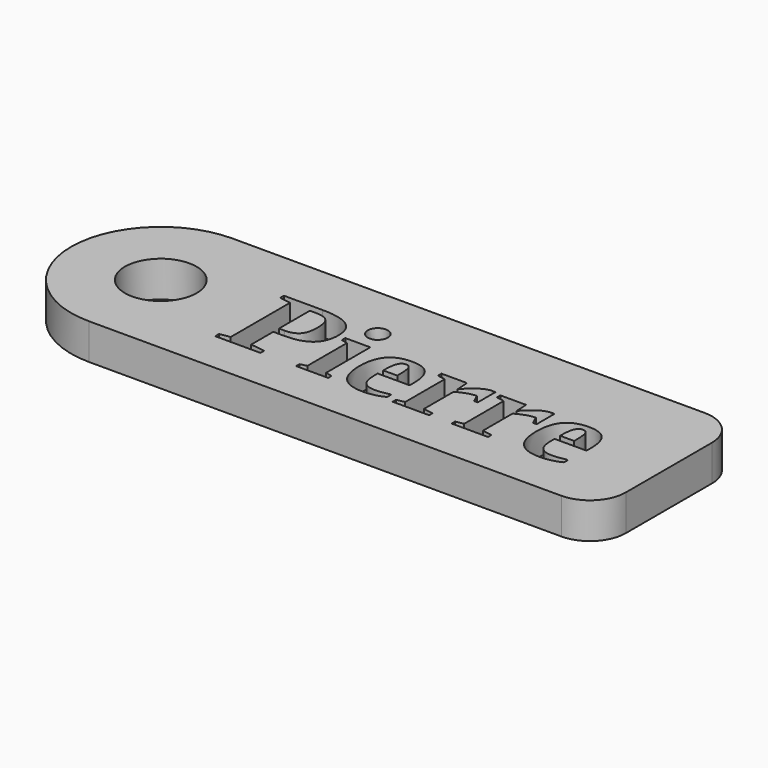
from build123d import *

# Parameters (mm, degrees)
F0_W         = 50
F0_H         = 15
F1_DEPTH     = 3
F3_D         = 6
F4_R         = 7.49999
F5_R         = 3
F6_TEXT_SIZE = 11.1111111111
F7_DEPTH     = 2


# Not quite as in the source:
# - a fillet or chamfer is up to 0.001 mm smaller than in the source, because OpenCascade refuses the exact size
# - Text() gives the source's letters only with a copy of the font that has no kerning and outlines rounded to 1/6400 em; it was checked with that copy


with BuildPart() as f1:
    # F0 (on Top) → F1 (new body)
    with BuildSketch(Plane.XY):
        with Locations((25, 7.5)):
            Rectangle(F0_W, F0_H)
    extrude(amount=F1_DEPTH)

    # F3 (through all)
    with Locations(Plane.XY.offset(3)):
        with Locations((7.5, 7.5)):
            Hole(F3_D / 2)

    # F4 (radius 7.5 in the source; OpenCascade refuses exactly that, so slightly less here)
    f4_edges = [f1.edges().sort_by_distance(p)[0] for p in [
        (0, 15, 1.5),
        (0, 0, 1.5),
    ]]
    fillet(f4_edges, radius=F4_R)

    # F5
    f5_edges = [f1.edges().sort_by_distance(p)[0] for p in [
        (50, 15, 1.5),
        (50, 0, 1.5),
    ]]
    fillet(f5_edges, radius=F5_R)

    # F6 (on face) → F7 (cut)
    with BuildSketch(Plane.XY.offset(3)):
        with Locations((14.9913194444, 3.5)):
            Text('Pierre', F6_TEXT_SIZE, font='Tinos', font_style=FontStyle.BOLD, text_align=(TextAlign.LEFT, TextAlign.BOTTOM))
    extrude(amount=-F7_DEPTH, mode=Mode.SUBTRACT)


solid = f1.part
